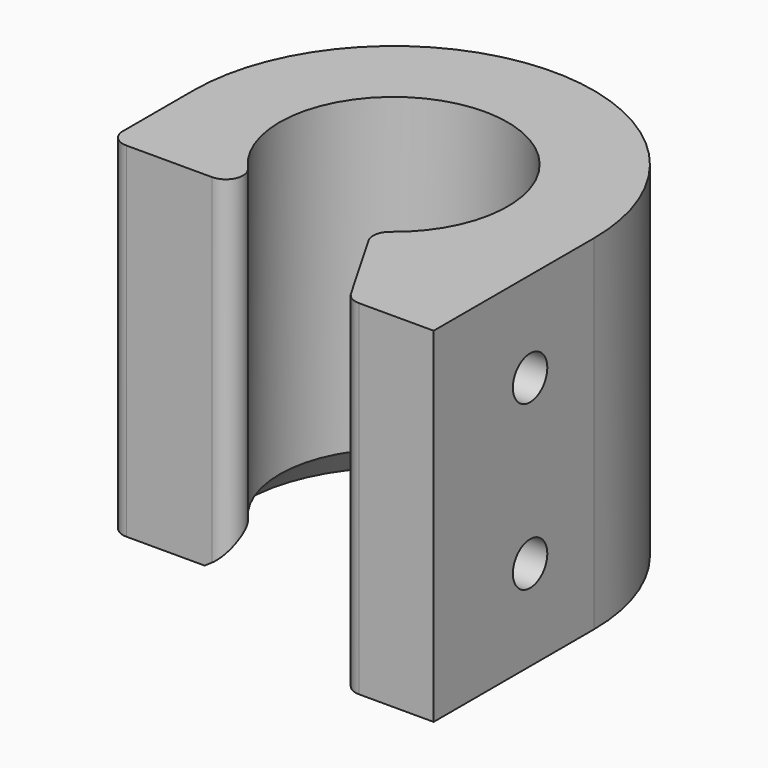
from build123d import *

# Parameters (mm, degrees)
F1_DEPTH    = 20
F2_R        = 1.25
F3_DEPTH    = 6
F4_T2_ANGLE = 359.64


# Not quite as in the source:
# - a fillet or chamfer that OpenCascade refuses, or shapes differently, is made with other operations: its cross-section is extruded or revolved along the edge and cut away or added
# - a feature names something its author has since deleted; it is built from what else it names


with BuildPart() as f1:
    # F0 (on Top) → F1 (new body)
    with BuildSketch(Plane.XY):
        with BuildLine():
            Line((11.625, -11.625), (11.625, 0))
            ThreePointArc((11.625, 0), (0, 11.625), (-11.625, 0))
            Line((-11.625, 0), (-11.625, -5.125))
            ThreePointArc((-11.625, -5.125), (-11.3321067812, -5.8321067812), (-10.625, -6.125))
            Line((-10.625, -6.125), (-5.6457948953, -6.125))
            ThreePointArc((-5.6457948953, -6.125), (-4.7314286811, -5.5298881651), (-4.9053627779, -4.4528688525))
            ThreePointArc((-4.9053627779, -4.4528688525), (0.5907863647, 6.598605646), (4.0363377793, -5.2534371921))
            ThreePointArc((4.0363377793, -5.2534371921), (3.6647499446, -5.8516258782), (3.7795709082, -6.5464088438))
            Line((3.7795709082, -6.5464088438), (6.4230217447, -11.125))
            ThreePointArc((6.4230217447, -11.125), (6.7890471485, -11.4910254038), (7.2890471485, -11.625))
            Line((7.2890471485, -11.625), (11.625, -11.625))
        make_face()
    extrude(amount=F1_DEPTH)

    # F2 (on face) → F3 (cut)
    with BuildSketch(Plane.YZ.offset(11.625)):
        with Locations((-4.625, 14.75)):
            Circle(F2_R)
        with Locations((-4.625, 5.25)):
            Circle(F2_R)
    extrude(amount=-F3_DEPTH, mode=Mode.SUBTRACT)

    # F4: chamfer of 2 on 1 edges, made by hand

    # F4_s1 → F4_t2 (revolve, cut)
    with BuildSketch(Plane(origin=(0, 0, 0), x_dir=(0, 0, 1), z_dir=(0.9957308794, -0.0923039315, 0))):
        Polygon((0, 8.625), (2, 6.625), (0, 6.625), align=None)
    revolve(axis=Axis((0, 0, 0), (0, 0, -1)), revolution_arc=F4_T2_ANGLE, mode=Mode.SUBTRACT)


solid = f1.part
